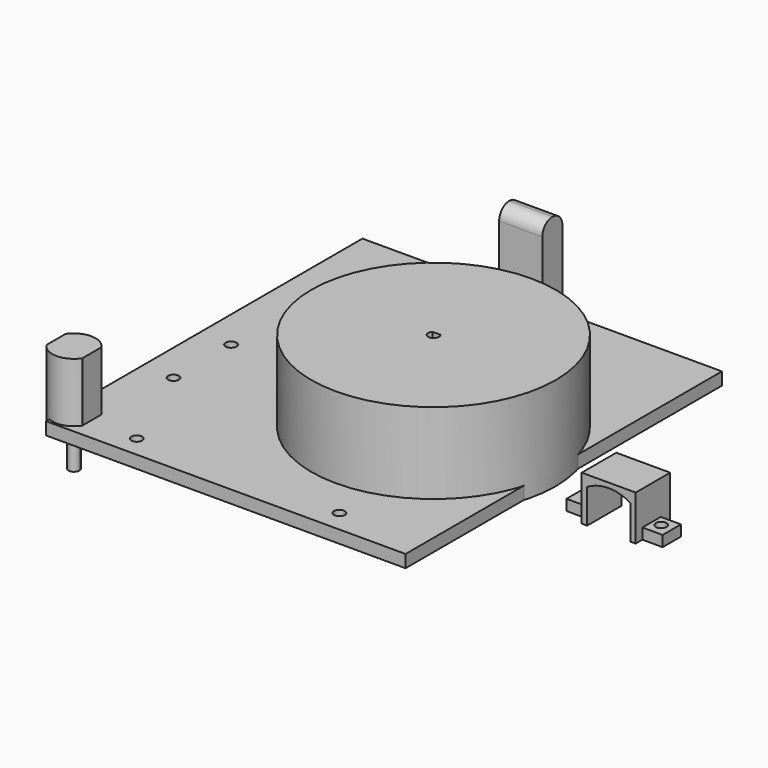
from build123d import *

# Parameters (mm, degrees)
F0_R      = 34
F1_DEPTH  = 26
F2_DEPTH  = 26
F4_DEPTH  = 20
F5_DEPTH  = 20
F6_DEPTH  = 20
F7_DEPTH  = 10
F8_W      = 100
F8_H      = 110
F8_R      = 1.5
F8_W_2    = 12
F8_H_2    = 7
F9_DEPTH  = 3.5
F10_DEPTH = 30.5
F11_R     = 3.5
F12_R     = 3.49999
F14_DEPTH = 12.5
F13_W     = 6.3024445623
F13_H     = 6.2478113687
F13_R     = 1.5
F15_DEPTH = 3
F13_W_2   = 5.6342094392
F13_H_2   = 6.382860709
F16_DEPTH = 3
F17_W     = 12
F17_H     = 10
F18_DEPTH = 25


# Not quite as in the source:
# - a fillet or chamfer is up to 0.001 mm smaller than in the source, because OpenCascade refuses the exact size


with BuildPart() as f1:
    # F0 (on Top) → F1 (new body)
    with BuildSketch(Plane.XY):
        Circle(F0_R)
        with BuildLine():
            ThreePointArc((1.1084163734, 1.0106498618), (1.3986823371, 0.5419296264), (1.5, 0))
            ThreePointArc((1.5, 0), (-0.5419296264, -1.3986823371), (-1.1084163734, 1.0106498618))
            ThreePointArc((-1.1084163734, 1.0106498618), (0, 1.5), (1.1084163734, 1.0106498618))
        make_face(mode=Mode.SUBTRACT)
    extrude(amount=F1_DEPTH)

    # F0 (on Top) → F2 (join)
    with BuildSketch(Plane.XY):
        with BuildLine():
            Line((-1.1084163734, 1.0106498618), (1.1084163734, 1.0106498618))
            ThreePointArc((1.1084163734, 1.0106498618), (0, 1.5), (-1.1084163734, 1.0106498618))
        make_face()
    extrude(amount=F2_DEPTH)


with BuildPart() as f4:
    # F3 (on Top) → F4 (new body)
    with BuildSketch(Plane.XY):
        with BuildLine():
            Line((-69.9148401618, -40.5942231864), (-69.9148401618, -47.2274727672))
            ThreePointArc((-69.9148401618, -47.2274727672), (-69.8523901158, -47.319748159), (-69.7882373342, -47.4108479768))
            Line((-69.7882373342, -47.4108479768), (-60.0414429894, -47.4108479768))
            ThreePointArc((-60.0414429894, -47.4108479768), (-59.9772902078, -47.319748159), (-59.9148401618, -47.2274727672))
            Line((-59.9148401618, -47.2274727672), (-59.9148401618, -40.5942231864))
            ThreePointArc((-59.9148401618, -40.5942231864), (-59.9772902078, -40.5019477946), (-60.0414429894, -40.4108479768))
            Line((-60.0414429894, -40.4108479768), (-69.7882373342, -40.4108479768))
            ThreePointArc((-69.7882373342, -40.4108479768), (-69.8523901158, -40.5019477946), (-69.9148401618, -40.5942231864))
        make_face()
        with BuildLine():
            ThreePointArc((-63.7968061731, -42.9108479768), (-63.5135816234, -43.3756148421), (-63.4148401618, -43.9108479768))
            ThreePointArc((-63.4148401618, -43.9108479768), (-65.4500732965, -45.3121065152), (-66.0328741506, -42.9108479768))
            ThreePointArc((-66.0328741506, -42.9108479768), (-64.9148401618, -42.4108479768), (-63.7968061731, -42.9108479768))
        make_face(mode=Mode.SUBTRACT)
    extrude(amount=F4_DEPTH)

    # F3 (on Top) → F5 (join)
    with BuildSketch(Plane.XY):
        with BuildLine():
            Line((-60.0414429894, -47.4108479768), (-69.7882373342, -47.4108479768))
            ThreePointArc((-69.7882373342, -47.4108479768), (-64.9148401618, -49.9108479768), (-60.0414429894, -47.4108479768))
        make_face()
        with BuildLine():
            Line((-66.0328741506, -42.9108479768), (-63.7968061731, -42.9108479768))
            ThreePointArc((-63.7968061731, -42.9108479768), (-64.9148401618, -42.4108479768), (-66.0328741506, -42.9108479768))
        make_face()
        with BuildLine():
            ThreePointArc((-66.0328741506, -42.9108479768), (-65.4500732965, -45.3121065152), (-63.4148401618, -43.9108479768))
            ThreePointArc((-63.4148401618, -43.9108479768), (-63.5135816234, -43.3756148421), (-63.7968061731, -42.9108479768))
            Line((-63.7968061731, -42.9108479768), (-66.0328741506, -42.9108479768))
        make_face()
    extrude(amount=F5_DEPTH)

    # F3 (on Top) → F6 (join)
    with BuildSketch(Plane.XY):
        with BuildLine():
            ThreePointArc((-60.0414429894, -40.4108479768), (-64.9148401618, -37.9108479768), (-69.7882373342, -40.4108479768))
            Line((-69.7882373342, -40.4108479768), (-60.0414429894, -40.4108479768))
        make_face()
    extrude(amount=F6_DEPTH)

    # F3 (on Top) → F7 (join)
    with BuildSketch(Plane.XY):
        with BuildLine():
            ThreePointArc((-66.0328741506, -42.9108479768), (-65.4500732965, -45.3121065152), (-63.4148401618, -43.9108479768))
            ThreePointArc((-63.4148401618, -43.9108479768), (-63.5135816234, -43.3756148421), (-63.7968061731, -42.9108479768))
            Line((-63.7968061731, -42.9108479768), (-66.0328741506, -42.9108479768))
        make_face()
    extrude(amount=-F7_DEPTH)


with BuildPart() as f9:
    # F8 (on Top) → F9 (new body)
    with BuildSketch(Plane.XY):
        with Locations((-17.3735144734, 4.4944389339)):
            Rectangle(F8_W, F8_H)
        with Locations((-46.8782410026, -44.6094162762)):
            Circle(F8_R, mode=Mode.SUBTRACT)
        with BuildLine():
            ThreePointArc((-58.4921389818, -15.7774437815), (-57.43147881, -16.2167836097), (-56.9921389818, -17.2774437815))
            ThreePointArc((-56.9921389818, -17.2774437815), (-59.5527991536, -18.3381039533), (-58.4921389818, -15.7774437815))
        make_face(mode=Mode.SUBTRACT)
        with BuildLine():
            ThreePointArc((-56.9921389818, 2.7225562185), (-57.43147881, 1.6618960467), (-58.4921389818, 1.2225562185))
            ThreePointArc((-58.4921389818, 1.2225562185), (-59.5527991536, 3.7832163903), (-56.9921389818, 2.7225562185))
        make_face(mode=Mode.SUBTRACT)
        with Locations((9.3834688887, -44.4461479783)):
            Circle(F8_R, mode=Mode.SUBTRACT)
        with BuildLine():
            ThreePointArc((24.3961110115, -17.2774437815), (21.8354508397, -18.3381039533), (22.8961110115, -15.7774437815))
            ThreePointArc((22.8961110115, -15.7774437815), (23.9567711833, -16.2167836097), (24.3961110115, -17.2774437815))
        make_face(mode=Mode.SUBTRACT)
        with BuildLine():
            ThreePointArc((24.3961110115, 2.7225562185), (23.9567711833, 1.6618960467), (22.8961110115, 1.2225562185))
            ThreePointArc((22.8961110115, 1.2225562185), (21.8354508397, 3.7832163903), (24.3961110115, 2.7225562185))
        make_face(mode=Mode.SUBTRACT)
        with Locations((-17.4279436469, 45.7378067076)):
            Circle(F8_R, mode=Mode.SUBTRACT)
        with Locations((0, 20.8121649921)):
            Circle(F8_R, mode=Mode.SUBTRACT)
        with Locations((-15.1569909006, 52.7596849799)):
            Rectangle(F8_W_2, F8_H_2, mode=Mode.SUBTRACT)
    extrude(amount=F9_DEPTH)

    # F8 (on Top) → F10 (join)
    with BuildSketch(Plane.XY):
        with Locations((-15.1569909006, 52.7596849799)):
            Rectangle(F8_W_2, F8_H_2)
    extrude(amount=F10_DEPTH)

    # F11
    f11_edges = [f9.edges().sort_by_distance(p)[0] for p in [
        (-15.156991, 49.259685, 30.5),
    ]]
    fillet(f11_edges, radius=F11_R)

    # F12 (radius 3.5 in the source; OpenCascade refuses exactly that, so slightly less here)
    f12_edges = [f9.edges().sort_by_distance(p)[0] for p in [
        (-15.156991, 56.259685, 30.5),
    ]]
    fillet(f12_edges, radius=F12_R)


with BuildPart() as f14:
    # F13 (on Top) → F14 (new body)
    with BuildSketch(Plane.XY):
        Polygon((64.406843558, 1.7756032334), (49.406843558, 1.7756032334), (49.406843558, -1.4032047475), (49.406843558, -7.6510161161), (49.406843558, -10.2243967666), (64.406843558, -10.2243967666), (64.406843558, -7.8880153596), (64.406843558, -1.5051546507), align=None)
    extrude(amount=F14_DEPTH)

    # F13 (on Top) → F15 (join)
    with BuildSketch(Plane.XY):
        with Locations((46.2556212768, -4.5271104318)):
            Rectangle(F13_W, F13_H)
        with Locations((46.8652057648, -4.4069956057)):
            Circle(F13_R, mode=Mode.SUBTRACT)
    extrude(amount=F15_DEPTH)

    # F13 (on Top) → F16 (join)
    with BuildSketch(Plane.XY):
        with Locations((67.2239482775, -4.6965850051)):
            Rectangle(F13_W_2, F13_H_2)
        with Locations((66.8652057648, -4.4403001666)):
            Circle(F13_R, mode=Mode.SUBTRACT)
    extrude(amount=F16_DEPTH)

    # F17 (on face) → F18 (cut)
    with BuildSketch(Plane.XZ.offset(10.2243967666)):
        with BuildLine():
            ThreePointArc((62.906843558, 9.5), (56.906843558, 11.1443961122), (50.906843558, 9.5))
            Line((50.906843558, 9.5), (62.906843558, 9.5))
        make_face()
        with Locations((56.906843558, 4.5)):
            Rectangle(F17_W, F17_H)
    extrude(amount=-F18_DEPTH, mode=Mode.SUBTRACT)


solid = Compound([f1.part, f4.part, f9.part, f14.part])
